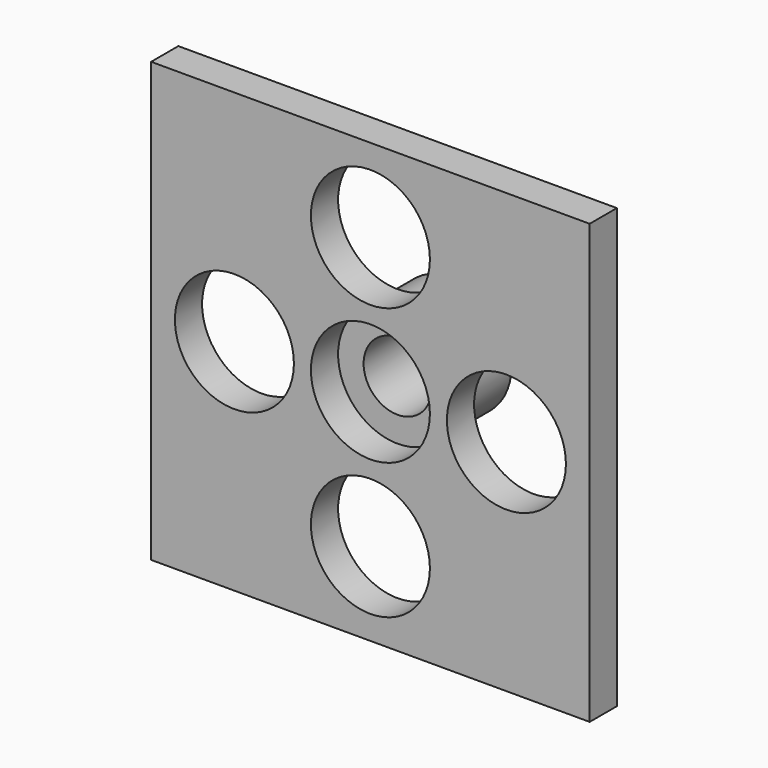
from build123d import *

# Parameters (mm, degrees)
F0_R     = 3.5
F0_R_2   = 2
F1_DEPTH = 4
F0_W     = 25.796212926
F0_H     = 25.796212926
F2_DEPTH = 2
F3_DEPTH = 2


# Not quite as in the source:
# - a feature names something its author has since deleted; it is built from what else it names


with BuildPart() as f1:
    # F0 (on Front) → F1 (new body)
    with BuildSketch(Plane.XZ):
        with Locations((0.3555135969, -0.4811176085)):
            Circle(F0_R)
        with Locations((0.3555135969, -0.4811176085)):
            Circle(F0_R_2, mode=Mode.SUBTRACT)
    extrude(amount=-F1_DEPTH)


with BuildPart() as f2:
    # F0 (on Front) → F2 (new body)
    with BuildSketch(Plane.XZ):
        with Locations((0.3555135969, -0.4811176085)):
            Rectangle(F0_W, F0_H)
        with Locations((0.3555135969, -8.4811176085)):
            Circle(F0_R, mode=Mode.SUBTRACT)
        with Locations((0.3555135969, -0.4811176085)):
            Circle(F0_R, mode=Mode.SUBTRACT)
        with Locations((-7.6444864031, -0.4811176085)):
            Circle(F0_R, mode=Mode.SUBTRACT)
        with Locations((0.3555135969, 7.5188823915)):
            Circle(F0_R, mode=Mode.SUBTRACT)
        with Locations((8.3555135969, -0.4811176085)):
            Circle(F0_R, mode=Mode.SUBTRACT)
    extrude(amount=F2_DEPTH)


with BuildPart() as f3:
    # F3 (new): a face of the model
    f3_faces = [f1.part.faces().sort_by_distance(p)[0] for p in [
        (-3.0454914538, 0, -0.4811176085),
    ]]
    extrude(f3_faces, amount=F3_DEPTH)


solid = Compound([f1.part, f2.part])
